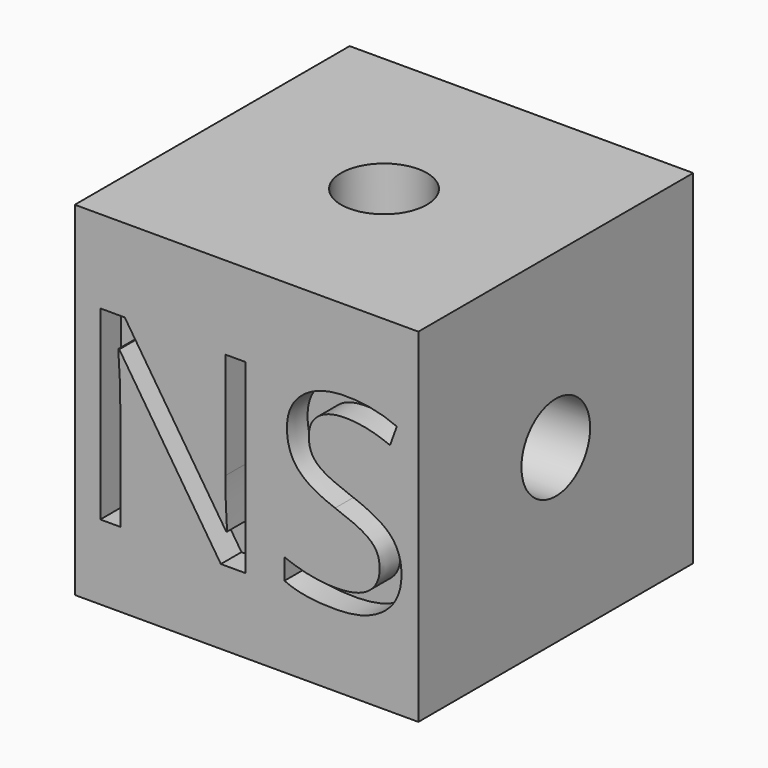
from build123d import *

# Parameters (mm, degrees)
F0_W         = 40
F0_H         = 40
F1_DEPTH     = 40
F2_R         = 5
F3_DEPTH     = 10
F4_R         = 5
F5_DEPTH     = 10
F6_TEXT_SIZE = 30.3102060147
F7_DEPTH     = 3
F8_R         = 5
F9_DEPTH     = 10
F10_R        = 5
F11_DEPTH    = 10
F12_R        = 5
F13_DEPTH    = 10


# Not quite as in the source:
# - Text() gives the source's letters only with a copy of the font that has no kerning and outlines rounded to 1/6400 em; it was checked with that copy


with BuildPart() as f1:
    # F0 (on Front) → F1 (new body)
    with BuildSketch(Plane.XZ):
        with Locations((20, 20)):
            Rectangle(F0_W, F0_H)
    extrude(amount=F1_DEPTH)

    # F2 (on face) → F3 (cut)
    with BuildSketch(Plane(origin=(0, 0, 0), x_dir=(0, -1, 0), z_dir=(-1, 0, 0))):
        with Locations((20, 20)):
            Circle(F2_R)
    extrude(amount=-F3_DEPTH, mode=Mode.SUBTRACT)

    # F4 (on face) → F5 (cut)
    with BuildSketch(Plane.YZ.offset(40)):
        with Locations((-20, 20)):
            Circle(F4_R)
    extrude(amount=-F5_DEPTH, mode=Mode.SUBTRACT)

    # F6 (on face) → F7 (cut)
    with BuildSketch(Plane.XZ.offset(40)):
        with Locations((0, 8.7059885753)):
            Text('NS', F6_TEXT_SIZE, font='Open Sans', text_align=(TextAlign.LEFT, TextAlign.BOTTOM))
    extrude(amount=-F7_DEPTH, mode=Mode.SUBTRACT)

    # F8 (on face) → F9 (cut)
    with BuildSketch(Plane.XY.offset(40)):
        with Locations((20, -20)):
            Circle(F8_R)
    extrude(amount=-F9_DEPTH, mode=Mode.SUBTRACT)

    # F10 (on face) → F11 (cut)
    with BuildSketch(Plane(origin=(0, 0, 0), x_dir=(1, 0, 0), z_dir=(0, 0, -1))):
        with Locations((20, 20)):
            Circle(F10_R)
    extrude(amount=-F11_DEPTH, mode=Mode.SUBTRACT)

    # F12 (on face) → F13 (cut)
    with BuildSketch(Plane(origin=(0, 0, 0), x_dir=(-1, 0, 0), z_dir=(0, 1, 0))):
        with Locations((-20, 20)):
            Circle(F12_R)
    extrude(amount=-F13_DEPTH, mode=Mode.SUBTRACT)


solid = f1.part
